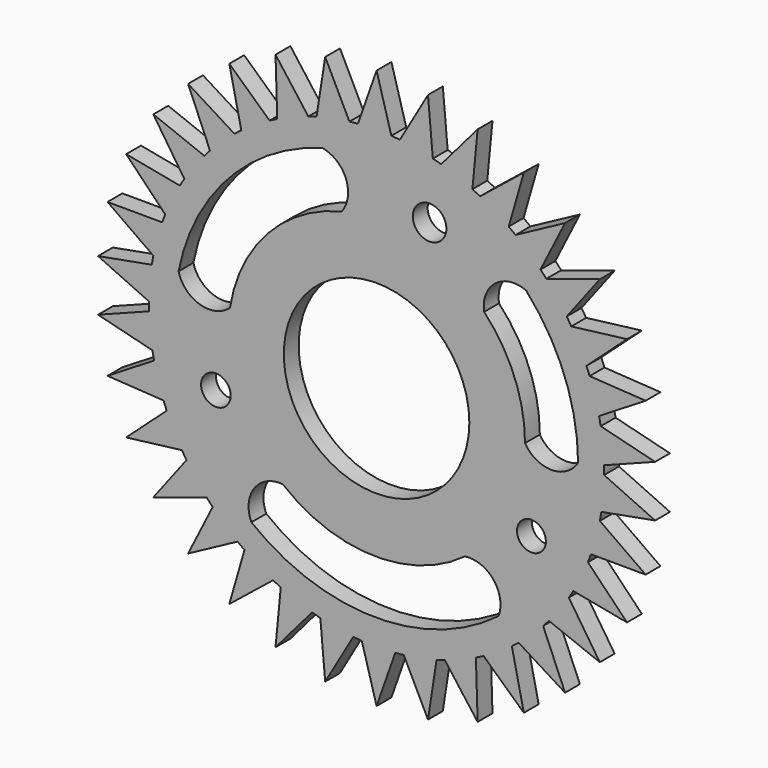
from build123d import *

# Parameters (mm, degrees)
F0_R     = 31.75
F0_R_2   = 5.0629734341
F0_R_3   = 5.7500073615
F0_R_4   = 4.9347024954
F1_DEPTH = 6.35


# Not quite as in the source:
# - a feature names something its author has since deleted; it is built from what else it names


with BuildPart() as f1:
    # F0 (on Front) → F1 (new body)
    with BuildSketch(Plane.XZ):
        with BuildLine():
            ThreePointArc((77.8839023703, -0.80358056), (77.8870114359, -0.4017956262), (77.8880478003, 0))
            ThreePointArc((77.8880478003, 0), (77.8807441552, 1.0666208171), (77.8588345898, 2.1330415979))
            ThreePointArc((77.8588345898, 2.1330415979), (77.4916211178, 7.8483531189), (76.7054384688, 13.5212314323))
            ThreePointArc((76.7054384688, 13.5212314323), (76.4369008567, 14.9648981809), (76.1411946094, 16.4032458249))
            ThreePointArc((76.1411946094, 16.4032458249), (74.7300479084, 21.953768008), (72.9148628583, 27.3855941052))
            ThreePointArc((72.9148628583, 27.3855941052), (72.3856245404, 28.7553360271), (71.8306575679, 30.1148571889))
            ThreePointArc((71.8306575679, 30.1148571889), (69.4236325463, 35.3115736581), (66.6412590449, 40.3173732161))
            ThreePointArc((66.6412590449, 40.3173732161), (65.8693425974, 41.5665453932), (65.0740136343, 42.80094321))
            ThreePointArc((65.0740136343, 42.80094321), (61.7530786424, 47.4668860189), (58.0982670821, 51.8761925375))
            ThreePointArc((58.0982670821, 51.8761925375), (57.1099591938, 52.9622559095), (56.101352214, 54.0294944442))
            ThreePointArc((56.101352214, 54.0294944442), (51.9795977099, 58.0057705066), (47.5768083151, 61.6684303408))
            ThreePointArc((47.5768083151, 61.6684303408), (46.4057646258, 62.554400322), (45.2182265303, 63.4181360464))
            ThreePointArc((45.2182265303, 63.4181360464), (40.4360139201, 66.5693380499), (35.4351784029, 69.3606237118))
            ThreePointArc((35.4351784029, 69.3606237118), (34.1212774009, 70.0163296572), (32.7952483753, 70.6471490871))
            ThreePointArc((32.7952483753, 70.6471490871), (27.5154301738, 72.865966627), (22.0868459901, 74.6908242313))
            ThreePointArc((22.0868459901, 74.6908242313), (20.6748309982, 75.0939368614), (19.2554673705, 75.4703581977))
            ThreePointArc((19.2554673705, 75.4703581977), (13.6578414541, 76.6812321038), (7.9863725273, 77.4775183134))
            ThreePointArc((7.9863725273, 77.4775183134), (6.5243280225, 77.6143101109), (5.0599645188, 77.7235147765))
            ThreePointArc((5.0599645188, 77.7235147765), (-0.6648486755, 77.8852101903), (-6.3860672734, 77.6258084333))
            ThreePointArc((-6.3860672734, 77.6258084333), (-7.8483531189, 77.4916211178), (-9.3078493559, 77.3298902787))
            ThreePointArc((-9.3078493559, 77.3298902787), (-14.9648981809, 76.4369008567), (-20.5410372122, 75.1306447489))
            ThreePointArc((-20.5410372122, 75.1306447489), (-21.953768008, 74.7300479084), (-23.3586955842, 74.3028891144))
            ThreePointArc((-23.3586955842, 74.3028891144), (-28.7553360271, 72.3856245404), (-33.9965067651, 70.0769970669))
            ThreePointArc((-33.9965067651, 70.0769970669), (-35.3115736581, 69.4236325463), (-36.6140894501, 68.7455921778))
            ThreePointArc((-36.6140894501, 68.7455921778), (-41.5665453932, 65.8693425974), (-46.2942660544, 62.6369612979))
            ThreePointArc((-46.2942660544, 62.6369612979), (-47.4668860189, 61.7530786424), (-48.6226344136, 60.8472465509))
            ThreePointArc((-48.6226344136, 60.8472465509), (-52.9622559095, 57.1099591938), (-57.015529637, 53.0638989366))
            ThreePointArc((-57.015529637, 53.0638989366), (-58.0057705066, 51.9795977099), (-58.9753938785, 50.8768209209))
            ThreePointArc((-58.9753938785, 50.8768209209), (-62.554400322, 46.4057646258), (-65.7951977405, 41.6838091401))
            ThreePointArc((-65.7951977405, 41.6838091401), (-66.5693380499, 40.4360139201), (-67.3198170381, 39.1738461744))
            ThreePointArc((-67.3198170381, 39.1738461744), (-70.0163296572, 34.1212774009), (-72.3342892975, 28.8842272176))
            ThreePointArc((-72.3342892975, 28.8842272176), (-72.865966627, 27.5154301738), (-73.3717445697, 26.1368530804))
            ThreePointArc((-73.3717445697, 26.1368530804), (-75.0939368614, 20.6748309982), (-76.410123388, 15.1010275801))
            ThreePointArc((-76.410123388, 15.1010275801), (-76.6812321038, 13.6578414541), (-76.9250853396, 12.2098008024))
            ThreePointArc((-76.9250853396, 12.2098008024), (-77.6143101109, 6.5243280225), (-77.8839023703, 0.80358056))
            ThreePointArc((-77.8839023703, 0.80358056), (-77.8852101903, -0.6648486755), (-77.8588345898, -2.1330415979))
            ThreePointArc((-77.8588345898, -2.1330415979), (-77.4916211178, -7.8483531189), (-76.7054384688, -13.5212314323))
            ThreePointArc((-76.7054384688, -13.5212314323), (-76.4369008567, -14.9648981809), (-76.1411946094, -16.4032458249))
            ThreePointArc((-76.1411946094, -16.4032458249), (-74.7300479084, -21.953768008), (-72.9148628583, -27.3855941052))
            ThreePointArc((-72.9148628583, -27.3855941052), (-72.3856245404, -28.7553360271), (-71.8306575679, -30.1148571889))
            ThreePointArc((-71.8306575679, -30.1148571889), (-69.4236325463, -35.3115736581), (-66.6412590449, -40.3173732161))
            ThreePointArc((-66.6412590449, -40.3173732161), (-65.8693425974, -41.5665453932), (-65.0740136343, -42.80094321))
            ThreePointArc((-65.0740136343, -42.80094321), (-61.7530786424, -47.4668860189), (-58.0982670821, -51.8761925375))
            ThreePointArc((-58.0982670821, -51.8761925375), (-57.1099591938, -52.9622559095), (-56.101352214, -54.0294944442))
            ThreePointArc((-56.101352214, -54.0294944442), (-51.9795977099, -58.0057705066), (-47.5768083151, -61.6684303408))
            ThreePointArc((-47.5768083151, -61.6684303408), (-46.4057646258, -62.554400322), (-45.2182265303, -63.4181360464))
            ThreePointArc((-45.2182265303, -63.4181360464), (-40.4360139201, -66.5693380499), (-35.4351784029, -69.3606237118))
            ThreePointArc((-35.4351784029, -69.3606237118), (-34.1212774009, -70.0163296572), (-32.7952483753, -70.6471490871))
            ThreePointArc((-32.7952483753, -70.6471490871), (-27.5154301738, -72.865966627), (-22.0868459901, -74.6908242313))
            ThreePointArc((-22.0868459901, -74.6908242313), (-20.6748309982, -75.0939368614), (-19.2554673705, -75.4703581977))
            ThreePointArc((-19.2554673705, -75.4703581977), (-13.6578414541, -76.6812321038), (-7.9863725273, -77.4775183134))
            ThreePointArc((-7.9863725273, -77.4775183134), (-6.5243280225, -77.6143101109), (-5.0599645188, -77.7235147765))
            ThreePointArc((-5.0599645188, -77.7235147765), (0.6648486755, -77.8852101903), (6.3860672734, -77.6258084333))
            ThreePointArc((6.3860672734, -77.6258084333), (7.8483531189, -77.4916211178), (9.3078493559, -77.3298902787))
            ThreePointArc((9.3078493559, -77.3298902787), (14.9648981809, -76.4369008567), (20.5410372122, -75.1306447489))
            ThreePointArc((20.5410372122, -75.1306447489), (21.953768008, -74.7300479084), (23.3586955842, -74.3028891144))
            ThreePointArc((23.3586955842, -74.3028891144), (28.7553360271, -72.3856245404), (33.9965067651, -70.0769970669))
            ThreePointArc((33.9965067651, -70.0769970669), (35.3115736581, -69.4236325463), (36.6140894501, -68.7455921778))
            ThreePointArc((36.6140894501, -68.7455921778), (41.5665453932, -65.8693425974), (46.2942660544, -62.6369612979))
            ThreePointArc((46.2942660544, -62.6369612979), (47.4668860189, -61.7530786424), (48.6226344136, -60.8472465509))
            ThreePointArc((48.6226344136, -60.8472465509), (52.9622559095, -57.1099591938), (57.015529637, -53.0638989366))
            ThreePointArc((57.015529637, -53.0638989366), (58.0057705066, -51.9795977099), (58.9753938785, -50.8768209209))
            ThreePointArc((58.9753938785, -50.8768209209), (62.554400322, -46.4057646258), (65.7951977405, -41.6838091401))
            ThreePointArc((65.7951977405, -41.6838091401), (66.5693380499, -40.4360139201), (67.3198170381, -39.1738461744))
            ThreePointArc((67.3198170381, -39.1738461744), (70.0163296572, -34.1212774009), (72.3342892975, -28.8842272176))
            ThreePointArc((72.3342892975, -28.8842272176), (72.865966627, -27.5154301738), (73.3717445697, -26.1368530804))
            ThreePointArc((73.3717445697, -26.1368530804), (75.0939368614, -20.6748309982), (76.410123388, -15.1010275801))
            ThreePointArc((76.410123388, -15.1010275801), (76.6812321038, -13.6578414541), (76.9250853396, -12.2098008024))
            ThreePointArc((76.9250853396, -12.2098008024), (77.6143101109, -6.5243280225), (77.8839023703, -0.80358056))
        make_face()
        with BuildLine():
            ThreePointArc((51.2159425895, 46.0695953976), (64.3505988888, 24.6760448542), (68.9653590458, 0))
            ThreePointArc((68.9653590458, 0), (68.9654635086, -0.0693316178), (68.9654983296, -0.1386633056))
            ThreePointArc((68.9654983296, -0.1386633056), (61.7929178431, -30.7768421885), (41.7658685149, -55.0474254387))
            ThreePointArc((41.7658685149, -55.0474254387), (-0.6698206342, -69.1587974533), (-42.8484053842, -54.2965795101))
            ThreePointArc((-42.8484053842, -54.2965795101), (-64.802911177, -24.0586707713), (-67.7810660452, 13.1899807892))
            ThreePointArc((-67.7810660452, 13.1899807892), (-50.6998117471, 46.7601152185), (-18.5376786599, 66.3642058449))
            ThreePointArc((-18.5376786599, 66.3642058449), (19.2250877509, 66.1360792806), (51.2159425895, 46.0695953976))
        make_face(mode=Mode.SUBTRACT)
        with BuildLine():
            ThreePointArc((30.2210684349, -40.8329159215), (45.3644699985, -22.8627395942), (50.8, 0))
            ThreePointArc((50.8, 0), (47.1768856411, 18.8409517065), (36.824351921, 34.9943867727))
            ThreePointArc((36.824351921, 34.9943867727), (14.3775405383, 48.7229548372), (-11.9264708635, 49.3801507971))
            ThreePointArc((-11.9264708635, 49.3801507971), (-37.3439360506, 34.4393734009), (-50.1823021287, 7.8978828214))
            ThreePointArc((-50.1823021287, 7.8978828214), (-47.4471108986, -18.1497015782), (-32.100039787, -39.3729278271))
            ThreePointArc((-32.100039787, -39.3729278271), (-1.1897582294, -50.7860657598), (30.2210684349, -40.8329159215))
        make_face()
        Circle(F0_R, mode=Mode.SUBTRACT)
        with BuildLine():
            ThreePointArc((-42.8484053842, -54.2965795101), (-41.8274002652, -43.6994925272), (-32.100039787, -39.3729278271))
            ThreePointArc((-32.100039787, -39.3729278271), (-47.4471108986, -18.1497015782), (-50.1823021287, 7.8978828214))
            ThreePointArc((-50.1823021287, 7.8978828214), (-60.4686343737, 5.5991089373), (-67.7810660452, 13.1899807892))
            ThreePointArc((-67.7810660452, 13.1899807892), (-64.802911177, -24.0586707713), (-42.8484053842, -54.2965795101))
        make_face()
        with Locations((-55.0011135638, -18.4467043728)):
            Circle(F0_R_2, mode=Mode.SUBTRACT)
        with BuildLine():
            ThreePointArc((-11.9264708635, 49.3801507971), (14.3775405383, 48.7229548372), (36.824351921, 34.9943867727))
            ThreePointArc((36.824351921, 34.9943867727), (40.6847909156, 44.8660930239), (51.2159425895, 46.0695953976))
            ThreePointArc((51.2159425895, 46.0695953976), (19.2250877509, 66.1360792806), (-18.5376786599, 66.3642058449))
            ThreePointArc((-18.5376786599, 66.3642058449), (-10.4717670738, 59.725174158), (-11.9264708635, 49.3801507971))
        make_face()
        with Locations((18.1432235986, 55.8405146003)):
            Circle(F0_R_3, mode=Mode.SUBTRACT)
        with BuildLine():
            ThreePointArc((68.9653590458, 0), (59.8826795229, -5.1335011671), (50.8, 0))
            ThreePointArc((50.8, 0), (45.3644699985, -22.8627395942), (30.2210684349, -40.8329159215))
            ThreePointArc((30.2210684349, -40.8329159215), (40.0179259308, -44.6715699098), (41.7658685149, -55.0474254387))
            ThreePointArc((41.7658685149, -55.0474254387), (61.7929178431, -30.7768421885), (68.9654983296, -0.1386633056))
            ThreePointArc((68.9654983296, -0.1386633056), (68.9654635086, -0.0693316178), (68.9653590458, 0))
        make_face()
        with Locations((53.001075983, -27.3040272295)):
            Circle(F0_R_4, mode=Mode.SUBTRACT)
        with BuildLine():
            ThreePointArc((-20.5410372122, 75.1306447489), (-14.9648981809, 76.4369008567), (-9.3078493559, 77.3298902787))
            Line((-9.3078493559, 77.3298902787), (-17.592676785, 94.1125083567))
            Line((-17.592676785, 94.1125083567), (-20.5410372122, 75.1306447489))
        make_face()
        with BuildLine():
            ThreePointArc((-6.3860672734, 77.6258084333), (-0.6648486755, 77.8852101903), (5.0599645188, 77.7235147765))
            Line((5.0599645188, 77.7235147765), (0, 95.7427099347))
            Line((0, 95.7427099347), (-6.3860672734, 77.6258084333))
        make_face()
        with BuildLine():
            ThreePointArc((7.9863725273, 77.4775183134), (13.6578414541, 76.6812321038), (19.2554673705, 75.4703581977))
            Line((19.2554673705, 75.4703581977), (17.592676785, 94.1125083567))
            Line((17.592676785, 94.1125083567), (7.9863725273, 77.4775183134))
        make_face()
        with BuildLine():
            ThreePointArc((22.0868459901, 74.6908242313), (27.5154301738, 72.865966627), (32.7952483753, 70.6471490871))
            Line((32.7952483753, 70.6471490871), (34.5862560621, 89.277418182))
            Line((34.5862560621, 89.277418182), (22.0868459901, 74.6908242313))
        make_face()
        with BuildLine():
            Line((-95.3342884131, -8.8340227762), (-76.7054384688, -13.5212314323))
            ThreePointArc((-76.7054384688, -13.5212314323), (-77.4916211178, -7.8483531189), (-77.8588345898, -2.1330415979))
            Line((-77.8588345898, -2.1330415979), (-95.3342884131, -8.8340227762))
        make_face()
        with BuildLine():
            ThreePointArc((-77.8839023703, 0.80358056), (-77.6143101109, 6.5243280225), (-76.9250853396, 12.2098008024))
            Line((-76.9250853396, 12.2098008024), (-95.3342884131, 8.8340227762))
            Line((-95.3342884131, 8.8340227762), (-77.8839023703, 0.80358056))
        make_face()
        with BuildLine():
            ThreePointArc((-76.410123388, 15.1010275801), (-75.0939368614, 20.6748309982), (-73.3717445697, 26.1368530804))
            Line((-73.3717445697, 26.1368530804), (-92.0877935621, 26.2012362783))
            Line((-92.0877935621, 26.2012362783), (-76.410123388, 15.1010275801))
        make_face()
        with BuildLine():
            ThreePointArc((-72.3342892975, 28.8842272176), (-70.0163296572, 34.1212774009), (-67.3198170381, 39.1738461744))
            Line((-67.3198170381, 39.1738461744), (-85.7053593484, 42.6761981039))
            Line((-85.7053593484, 42.6761981039), (-72.3342892975, 28.8842272176))
        make_face()
        with BuildLine():
            ThreePointArc((-65.7951977405, 41.6838091401), (-62.554400322, 46.4057646258), (-58.9753938785, 50.8768209209))
            Line((-58.9753938785, 50.8768209209), (-76.4043319144, 57.6978731875))
            Line((-76.4043319144, 57.6978731875), (-65.7951977405, 41.6838091401))
        make_face()
        with BuildLine():
            ThreePointArc((-57.015529637, 53.0638989366), (-52.9622559095, 57.1099591938), (-48.6226344136, 60.8472465509))
            Line((-48.6226344136, 60.8472465509), (-64.5014465939, 70.7547164006))
            Line((-64.5014465939, 70.7547164006), (-57.015529637, 53.0638989366))
        make_face()
        with BuildLine():
            ThreePointArc((-46.2942660544, 62.6369612979), (-41.5665453932, 65.8693425974), (-36.6140894501, 68.7455921778))
            Line((-36.6140894501, 68.7455921778), (-50.4020418707, 81.4020926077))
            Line((-50.4020418707, 81.4020926077), (-46.2942660544, 62.6369612979))
        make_face()
        with BuildLine():
            ThreePointArc((-33.9965067651, 70.0769970669), (-28.7553360271, 72.3856245404), (-23.3586955842, 74.3028891144))
            Line((-23.3586955842, 74.3028891144), (-34.5862560621, 89.277418182))
            Line((-34.5862560621, 89.277418182), (-33.9965067651, 70.0769970669))
        make_face()
        with BuildLine():
            ThreePointArc((35.4351784029, 69.3606237118), (40.4360139201, 66.5693380499), (45.2182265303, 63.4181360464))
            Line((45.2182265303, 63.4181360464), (50.4020418707, 81.4020926077))
            Line((50.4020418707, 81.4020926077), (35.4351784029, 69.3606237118))
        make_face()
        with BuildLine():
            ThreePointArc((47.5768083151, 61.6684303408), (51.9795977099, 58.0057705066), (56.101352214, 54.0294944442))
            Line((56.101352214, 54.0294944442), (64.5014465939, 70.7547164006))
            Line((64.5014465939, 70.7547164006), (47.5768083151, 61.6684303408))
        make_face()
        with BuildLine():
            ThreePointArc((58.0982670821, 51.8761925375), (61.7530786424, 47.4668860189), (65.0740136343, 42.80094321))
            Line((65.0740136343, 42.80094321), (76.4043319144, 57.6978731875))
            Line((76.4043319144, 57.6978731875), (58.0982670821, 51.8761925375))
        make_face()
        with BuildLine():
            ThreePointArc((66.6412590449, 40.3173732161), (69.4236325463, 35.3115736581), (71.8306575679, 30.1148571889))
            Line((71.8306575679, 30.1148571889), (85.7053593484, 42.6761981039))
            Line((85.7053593484, 42.6761981039), (66.6412590449, 40.3173732161))
        make_face()
        with BuildLine():
            ThreePointArc((72.9148628583, 27.3855941052), (74.7300479084, 21.953768008), (76.1411946094, 16.4032458249))
            Line((76.1411946094, 16.4032458249), (92.0877935621, 26.2012362783))
            Line((92.0877935621, 26.2012362783), (72.9148628583, 27.3855941052))
        make_face()
        with BuildLine():
            ThreePointArc((76.7054384688, 13.5212314323), (77.4916211178, 7.8483531189), (77.8588345898, 2.1330415979))
            Line((77.8588345898, 2.1330415979), (95.3342884131, 8.8340227762))
            Line((95.3342884131, 8.8340227762), (76.7054384688, 13.5212314323))
        make_face()
        with BuildLine():
            Line((95.3342884131, -8.8340227762), (77.8839023703, -0.80358056))
            ThreePointArc((77.8839023703, -0.80358056), (77.6143101109, -6.5243280225), (76.9250853396, -12.2098008024))
            Line((76.9250853396, -12.2098008024), (95.3342884131, -8.8340227762))
        make_face()
        with BuildLine():
            Line((85.7053593484, -42.6761981039), (72.3342892975, -28.8842272176))
            ThreePointArc((72.3342892975, -28.8842272176), (70.0163296572, -34.1212774009), (67.3198170381, -39.1738461744))
            Line((67.3198170381, -39.1738461744), (85.7053593484, -42.6761981039))
        make_face()
        with BuildLine():
            Line((92.0877935621, -26.2012362783), (76.410123388, -15.1010275801))
            ThreePointArc((76.410123388, -15.1010275801), (75.0939368614, -20.6748309982), (73.3717445697, -26.1368530804))
            Line((73.3717445697, -26.1368530804), (92.0877935621, -26.2012362783))
        make_face()
        with BuildLine():
            Line((76.4043319144, -57.6978731875), (65.7951977405, -41.6838091401))
            ThreePointArc((65.7951977405, -41.6838091401), (62.554400322, -46.4057646258), (58.9753938785, -50.8768209209))
            Line((58.9753938785, -50.8768209209), (76.4043319144, -57.6978731875))
        make_face()
        with BuildLine():
            Line((64.5014465939, -70.7547164006), (57.015529637, -53.0638989366))
            ThreePointArc((57.015529637, -53.0638989366), (52.9622559095, -57.1099591938), (48.6226344136, -60.8472465509))
            Line((48.6226344136, -60.8472465509), (64.5014465939, -70.7547164006))
        make_face()
        with BuildLine():
            Line((34.5862560621, -89.277418182), (33.9965067651, -70.0769970669))
            ThreePointArc((33.9965067651, -70.0769970669), (28.7553360271, -72.3856245404), (23.3586955842, -74.3028891144))
            Line((23.3586955842, -74.3028891144), (34.5862560621, -89.277418182))
        make_face()
        with BuildLine():
            Line((17.592676785, -94.1125083567), (20.5410372122, -75.1306447489))
            ThreePointArc((20.5410372122, -75.1306447489), (14.9648981809, -76.4369008567), (9.3078493559, -77.3298902787))
            Line((9.3078493559, -77.3298902787), (17.592676785, -94.1125083567))
        make_face()
        with BuildLine():
            Line((0, -95.7427099347), (6.3860672734, -77.6258084333))
            ThreePointArc((6.3860672734, -77.6258084333), (0.6648486755, -77.8852101903), (-5.0599645188, -77.7235147765))
            Line((-5.0599645188, -77.7235147765), (0, -95.7427099347))
        make_face()
        with BuildLine():
            Line((-34.5862560621, -89.277418182), (-22.0868459901, -74.6908242313))
            ThreePointArc((-22.0868459901, -74.6908242313), (-27.5154301738, -72.865966627), (-32.7952483753, -70.6471490871))
            Line((-32.7952483753, -70.6471490871), (-34.5862560621, -89.277418182))
        make_face()
        with BuildLine():
            Line((-50.4020418707, -81.4020926077), (-35.4351784029, -69.3606237118))
            ThreePointArc((-35.4351784029, -69.3606237118), (-40.4360139201, -66.5693380499), (-45.2182265303, -63.4181360464))
            Line((-45.2182265303, -63.4181360464), (-50.4020418707, -81.4020926077))
        make_face()
        with BuildLine():
            Line((-64.5014465939, -70.7547164006), (-47.5768083151, -61.6684303408))
            ThreePointArc((-47.5768083151, -61.6684303408), (-51.9795977099, -58.0057705066), (-56.101352214, -54.0294944442))
            Line((-56.101352214, -54.0294944442), (-64.5014465939, -70.7547164006))
        make_face()
        with BuildLine():
            Line((-92.0877935621, -26.2012362783), (-72.9148628583, -27.3855941052))
            ThreePointArc((-72.9148628583, -27.3855941052), (-74.7300479084, -21.953768008), (-76.1411946094, -16.4032458249))
            Line((-76.1411946094, -16.4032458249), (-92.0877935621, -26.2012362783))
        make_face()
        with BuildLine():
            Line((50.4020418707, -81.4020926077), (46.2942660544, -62.6369612979))
            ThreePointArc((46.2942660544, -62.6369612979), (41.5665453932, -65.8693425974), (36.6140894501, -68.7455921778))
            Line((36.6140894501, -68.7455921778), (50.4020418707, -81.4020926077))
        make_face()
        with BuildLine():
            Line((-17.592676785, -94.1125083567), (-7.9863725273, -77.4775183134))
            ThreePointArc((-7.9863725273, -77.4775183134), (-13.6578414541, -76.6812321038), (-19.2554673705, -75.4703581977))
            Line((-19.2554673705, -75.4703581977), (-17.592676785, -94.1125083567))
        make_face()
        with BuildLine():
            Line((-76.4043319144, -57.6978731875), (-58.0982670821, -51.8761925375))
            ThreePointArc((-58.0982670821, -51.8761925375), (-61.7530786424, -47.4668860189), (-65.0740136343, -42.80094321))
            Line((-65.0740136343, -42.80094321), (-76.4043319144, -57.6978731875))
        make_face()
        with BuildLine():
            Line((-85.7053593484, -42.6761981039), (-66.6412590449, -40.3173732161))
            ThreePointArc((-66.6412590449, -40.3173732161), (-69.4236325463, -35.3115736581), (-71.8306575679, -30.1148571889))
            Line((-71.8306575679, -30.1148571889), (-85.7053593484, -42.6761981039))
        make_face()
    extrude(amount=F1_DEPTH)


solid = f1.part
